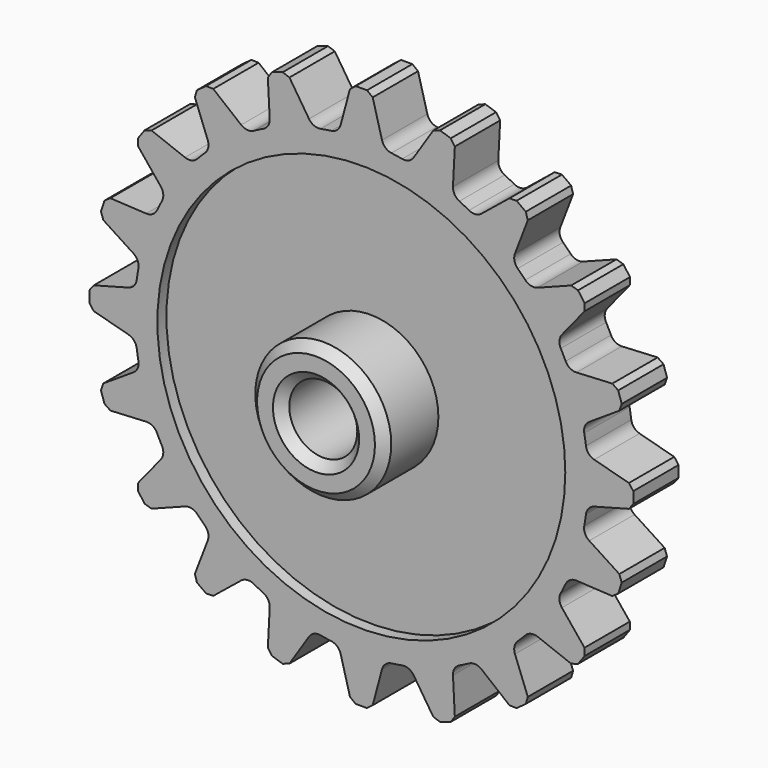
from build123d import *

# Parameters (mm, degrees)
F0_R            = 100
F1_DEPTH        = 25
F3_DEPTH        = 25
F3_COPIES_COUNT = 20
F4_SIZE         = 2
F5_R            = 5
F6_R            = 90
F7_DEPTH        = 5
F8_R            = 30
F9_DEPTH        = 30
F10_R           = 15
F11_DEPTH       = 50.001
F12_SIZE        = 4


# Not quite as in the source:
# - a pattern or mirror of a feature is missing from the dataset's text; its kind, count and spacing are read off the source's solid


with BuildPart() as f1:
    # F0 (on Front) → F1 (new body)
    with BuildSketch(Plane.XZ):
        Circle(F0_R)
    extrude(amount=F1_DEPTH)

    # F2 (on face) → F3 (join)
    with BuildSketch(Plane(origin=(0, 0, 0), x_dir=(-1, 0, 0), z_dir=(0, 1, 0))):
        with BuildLine():
            Line((4.5, 120), (-4.5, 120))
            Line((-4.5, 120), (-9.9931095726, 99.4994359837))
            ThreePointArc((-9.9931095726, 99.4994359837), (0, 100), (9.9931095726, 99.4994359837))
            Line((9.9931095726, 99.4994359837), (4.5, 120))
        make_face()
        with BuildLine():
            ThreePointArc((9.9931095726, 99.4994359837), (0, 100), (-9.9931095726, 99.4994359837))
            Line((-9.9931095726, 99.4994359837), (9.9931095726, 99.4994359837))
        make_face()
    f3 = extrude(amount=-F3_DEPTH)

    # F3_copies: F3 ×20 about axis
    f3_copies_axis = Axis((0, 0, 0), (0, 1, 0))
    for i in range(1, F3_COPIES_COUNT):
        add(f3.rotate(f3_copies_axis, i * 360 / F3_COPIES_COUNT))

    # F4
    f4_edges = [f1.edges().sort_by_distance(p)[0] for p in [
        (-4.5, -12.5, 120),
        (4.5, -12.5, 120),
        (-32.802285, -12.5, 115.517358),
        (32.802285, -12.5, 115.517358),
        (41.361794, -12.5, 112.736205),
        (66.893654, -12.5, 99.727073),
        (74.174807, -12.5, 94.437006),
        (94.437006, -12.5, 74.174807),
        (99.727073, -12.5, 66.893654),
        (112.736205, -12.5, 41.361794),
        (115.517358, -12.5, 32.802285),
        (120, -12.5, 4.5),
        (120, -12.5, -4.5),
        (115.517358, -12.5, -32.802285),
        (112.736205, -12.5, -41.361794),
        (99.727073, -12.5, -66.893654),
        (94.437006, -12.5, -74.174807),
        (74.174807, -12.5, -94.437006),
        (66.893654, -12.5, -99.727073),
        (41.361794, -12.5, -112.736205),
        (32.802285, -12.5, -115.517358),
        (4.5, -12.5, -120),
        (-4.5, -12.5, -120),
        (-32.802285, -12.5, -115.517358),
        (-41.361794, -12.5, -112.736205),
        (-66.893654, -12.5, -99.727073),
        (-74.174807, -12.5, -94.437006),
        (-94.437006, -12.5, -74.174807),
        (-99.727073, -12.5, -66.893654),
        (-112.736205, -12.5, -41.361794),
        (-115.517358, -12.5, -32.802285),
        (-120, -12.5, -4.5),
        (-120, -12.5, 4.5),
        (-115.517358, -12.5, 32.802285),
        (-112.736205, -12.5, 41.361794),
        (-99.727073, -12.5, 66.893654),
        (-94.437006, -12.5, 74.174807),
        (-74.174807, -12.5, 94.437006),
        (-66.893654, -12.5, 99.727073),
        (-41.361794, -12.5, 112.736205),
    ]]
    chamfer(f4_edges, length=F4_SIZE)

    # F5
    f5_edges = [f1.edges().sort_by_distance(p)[0] for p in [
        (-9.99311, -12.5, 99.499436),
        (9.99311, -12.5, 99.499436),
        (-21.243005, -12.5, 97.717628),
        (21.243005, -12.5, 97.717628),
        (-40.251029, -12.5, 91.541546),
        (-50.399706, -12.5, 86.370537),
        (40.251029, -12.5, 91.541546),
        (50.399706, -12.5, 86.370537),
        (-66.568897, -12.5, 74.622932),
        (-74.622932, -12.5, 66.568897),
        (66.568897, -12.5, 74.622932),
        (74.622932, -12.5, 66.568897),
        (-86.370537, -12.5, 50.399706),
        (-91.541546, -12.5, 40.251029),
        (86.370537, -12.5, 50.399706),
        (91.541546, -12.5, 40.251029),
        (-97.717628, -12.5, 21.243005),
        (-99.499436, -12.5, 9.99311),
        (97.717628, -12.5, 21.243005),
        (99.499436, -12.5, 9.99311),
        (-99.499436, -12.5, -9.99311),
        (-97.717628, -12.5, -21.243005),
        (99.499436, -12.5, -9.99311),
        (97.717628, -12.5, -21.243005),
        (-91.541546, -12.5, -40.251029),
        (-86.370537, -12.5, -50.399706),
        (91.541546, -12.5, -40.251029),
        (86.370537, -12.5, -50.399706),
        (-74.622932, -12.5, -66.568897),
        (-66.568897, -12.5, -74.622932),
        (74.622932, -12.5, -66.568897),
        (66.568897, -12.5, -74.622932),
        (-50.399706, -12.5, -86.370537),
        (-40.251029, -12.5, -91.541546),
        (50.399706, -12.5, -86.370537),
        (40.251029, -12.5, -91.541546),
        (-21.243005, -12.5, -97.717628),
        (-9.99311, -12.5, -99.499436),
        (21.243005, -12.5, -97.717628),
        (9.99311, -12.5, -99.499436),
    ]]
    fillet(f5_edges, radius=F5_R)

    # F6 (on face) → F7 (cut)
    with BuildSketch(Plane.XZ.offset(25)):
        Circle(F6_R)
    extrude(amount=-F7_DEPTH, mode=Mode.SUBTRACT)

    # F8 (on face) → F9 (join)
    with BuildSketch(Plane.XZ.offset(20)):
        Circle(F8_R)
    extrude(amount=F9_DEPTH)

    # F10 (on face) → F11 (cut, through all)
    with BuildSketch(Plane.XZ.offset(50)):
        Circle(F10_R)
    extrude(amount=-F11_DEPTH, mode=Mode.SUBTRACT)

    # F12
    f12_edges = [f1.edges().sort_by_distance(p)[0] for p in [
        (-15, -50, 0),
        (-30, -50, 0),
    ]]
    chamfer(f12_edges, length=F12_SIZE)


solid = f1.part
